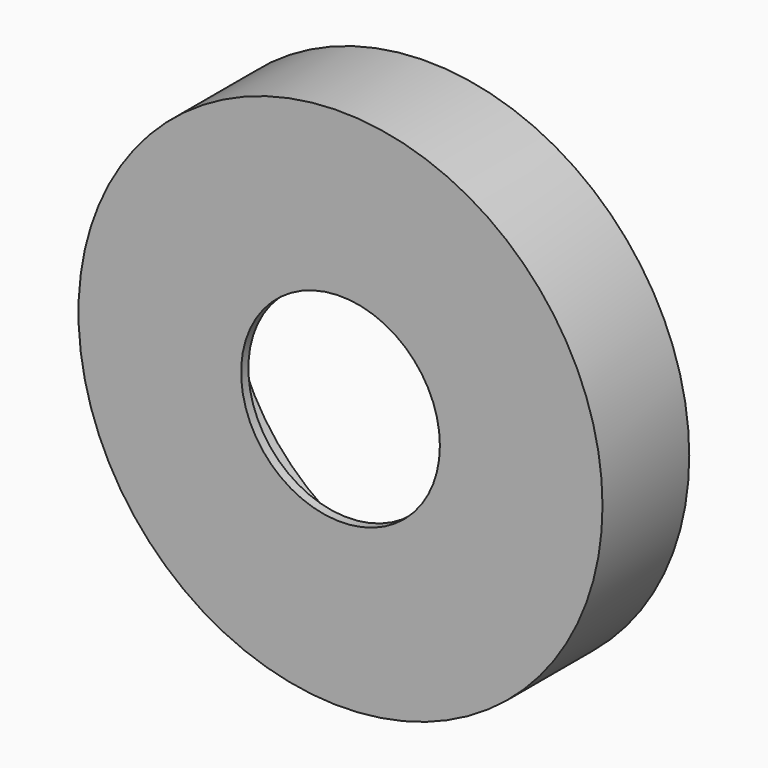
from build123d import *
from build123d import SkipClean  # not in build123d's __all__

# Parameters (mm, degrees)
F0_R     = 5.8
F1_DEPTH = 1.8
F2_R     = 5.8
F2_R_2   = 4.7
F3_DEPTH = 0.4
F4_R     = 4.7
F5_DEPTH = 1.8
F6_R     = 5.8
F6_R_2   = 4.7
F6_R_3   = 2.2
F7_DEPTH = 0.2
F8_R     = 5
F8_R_2   = 4.7
F9_DEPTH = 0.4


# Not quite as in the source:
# - a feature names something its author has since deleted; it is built from what else it names


with BuildPart() as f1:
    # F0 (on Front) → F1 (new body)
    with BuildSketch(Plane.XZ):
        Circle(F0_R)
    extrude(amount=F1_DEPTH)

    # F2 (on face) → F3 (join)
    with BuildSketch(Plane.XZ.offset(1.8)):
        Circle(F2_R)
        Circle(F2_R_2, mode=Mode.SUBTRACT)
    extrude(amount=F3_DEPTH)

    # F4 (on face) → F5 (cut)
    with BuildSketch(Plane.XZ.offset(1.8)):
        Circle(F4_R)
    extrude(amount=-F5_DEPTH, mode=Mode.SUBTRACT)

    # F6 (on face) → F7 (join)
    with BuildSketch(Plane.XZ.offset(2.2)):
        Circle(F6_R)
        Circle(F6_R_2, mode=Mode.SUBTRACT)
        Circle(F6_R_2)
        Circle(F6_R_3, mode=Mode.SUBTRACT)
    extrude(amount=F7_DEPTH)

    # F8 (on face) → F9 (join)
    with BuildSketch(Plane(origin=(0, 0, 0), x_dir=(-1, 0, 0), z_dir=(0, 1, 0))):
        Circle(F8_R)
        Circle(F8_R_2, mode=Mode.SUBTRACT)
    with SkipClean():  # cleaning this boolean's faces spoils the solid; the shape is the same uncleaned
        extrude(amount=F9_DEPTH)


solid = f1.part
